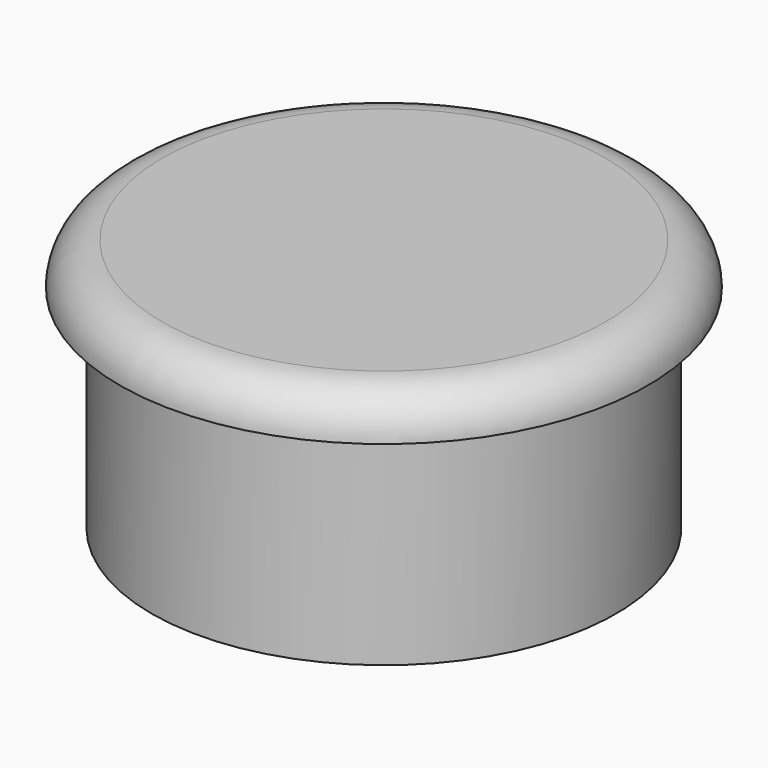
from build123d import *

# Parameters (mm, degrees)
F2_R = 1.99999


# Not quite as in the source:
# - a fillet or chamfer is up to 0.001 mm smaller than in the source, because OpenCascade refuses the exact size


with BuildPart() as f1:
    # F0 (on Front) → F1 (revolve)
    with BuildSketch(Plane.XZ):
        Polygon((0, 7.2039468596), (0, 10.2039468596), (-12.5, 10.2039468596), (-12.5, 8.2039468596), (-11, 8.2039468596), (-11, -1.7960531404), (-9, -1.853223308), (-9, 7.2039468596), align=None)
    revolve(axis=Axis((0, 0, 8.7039468596), (0, 0, -1)))

    # F2 (radius 2 in the source; OpenCascade refuses exactly that, so slightly less here)
    f2_edges = [f1.edges().sort_by_distance(p)[0] for p in [
        (12.5, 0, 10.203947),
    ]]
    fillet(f2_edges, radius=F2_R)


solid = f1.part
